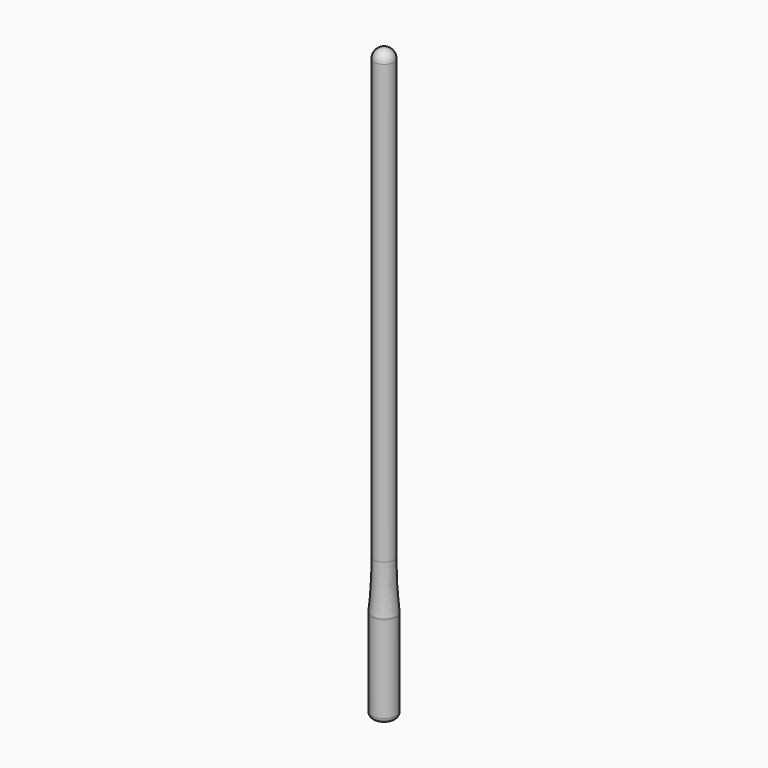
from build123d import *

# Parameters (mm, degrees)
F0_R     = 2.54
F1_DEPTH = 152.4
F2_R     = 2.54
F0_R_2   = 3.175
F3_DEPTH = 25.4
F5_R     = 127
F6_R     = 1.27


# Not quite as in the source:
# - a fillet or chamfer that OpenCascade refuses, or shapes differently, is made with other operations: its cross-section is extruded or revolved along the edge and cut away or added


with BuildPart() as f1:
    # F0 (on Top) → F1 (new body)
    with BuildSketch(Plane.XY):
        Circle(F0_R)
    extrude(amount=F1_DEPTH)

    # F2
    f2_edges = [f1.edges().sort_by_distance(p)[0] for p in [
        (-2.54, 0, 152.4),
    ]]
    fillet(f2_edges, radius=F2_R)

    # F0 (on Top) → F3 (join)
    with BuildSketch(Plane.XY):
        Circle(F0_R_2)
        Circle(F0_R, mode=Mode.SUBTRACT)
    extrude(amount=F3_DEPTH)

    # F4: fillet of radius 2.54 on 1 edges, made by hand

    # F4_s1 → F4_t2 (revolve, cut)
    with BuildSketch(Plane.XZ):
        with BuildLine():
            ThreePointArc((2.54, 25.4), (3.0109524406, 24.6179735296), (3.175, 23.7199479175))
            Line((3.175, 23.7199479175), (3.175, 25.4))
            Line((3.175, 25.4), (2.54, 25.4))
        make_face()
    revolve(axis=Axis((0, 0, 25.4), (0, 0, 1)), mode=Mode.SUBTRACT)

    # F5
    f5_edges = [f1.edges().sort_by_distance(p)[0] for p in [
        (-2.54, 0, 25.4),
    ]]
    fillet(f5_edges, radius=F5_R)

    # F6
    f6_edges = [f1.edges().sort_by_distance(p)[0] for p in [
        (-3.175, 0, 0),
    ]]
    fillet(f6_edges, radius=F6_R)


solid = f1.part
